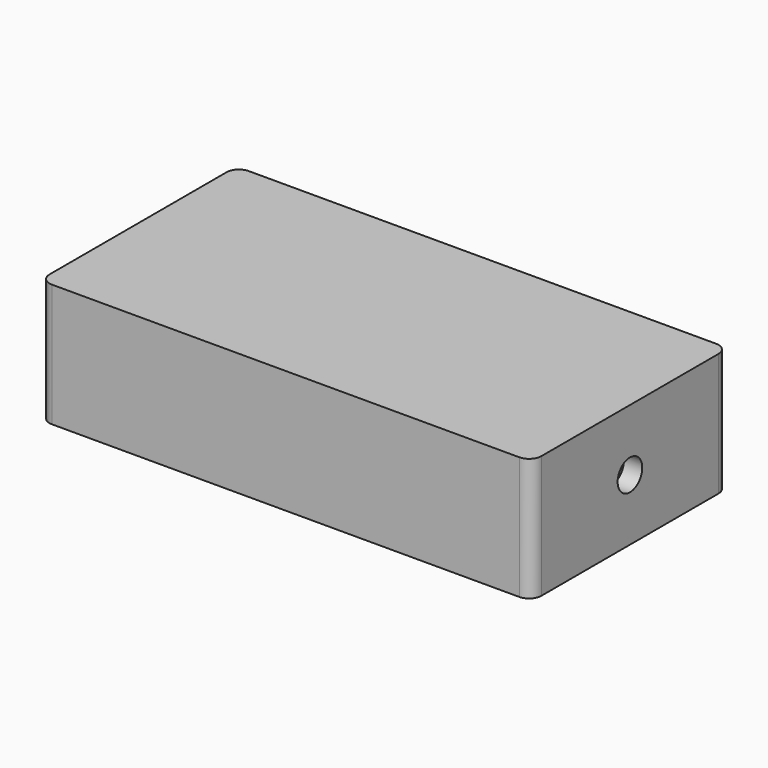
from build123d import *

# Parameters (mm, degrees)
F0_W          = 101.6
F0_H          = 50.8
F1_DEPTH      = 25.4
F2_T          = -3.81
F4_D          = 6.35
F4_DEPTH      = 12.7
F4_TIP        = 1.9077324654
F5_TEXT_SIZE  = 26.9125694306
F6_DEPTH      = 1.778
F7_W          = 93.98
F7_H          = 43.18
F7_W_2        = 88.9
F7_H_2        = 38.1
F8_DEPTH      = 21.59
F8_DEPTH_BACK = 2.54
F9_R          = 1.27
F10_R         = 2.54
F11_R         = 2.54


# Not quite as in the source:
# - Text() gives the source's letters only with a copy of the font that has no kerning and outlines rounded to 1/6400 em; it was checked with that copy


with BuildPart() as f1:
    # F0 (on Top) → F1 (new body)
    with BuildSketch(Plane.XY):
        with Locations((-25.4740342498, -0.3589369392)):
            Rectangle(F0_W, F0_H)
    extrude(amount=F1_DEPTH)

    # F2
    f2_openings = [f1.faces().sort_by_distance(p)[0] for p in [
        (-25.474034, -0.358937, 0),
    ]]
    offset(amount=F2_T, openings=f2_openings)

    # F4
    with Locations(Plane.YZ.offset(25.3259657502)):
        with Locations((-0.3589369392, 12.7)):
            Hole(F4_D / 2, depth=F4_DEPTH)
            with Locations((0, 0, -(F4_DEPTH + F4_TIP / 2))):  # 118° drill point
                Cone(0, F4_D / 2, F4_TIP, mode=Mode.SUBTRACT)

    # F5 (on face) → F6 (cut)
    with BuildSketch(Plane(origin=(0, 0, 21.59), x_dir=(1, 0, 0), z_dir=(0, 0, -1))):
        with Locations((-52.9090445489, -11.15504466)):
            Text('BOX', F5_TEXT_SIZE, font='Open Sans', text_align=(TextAlign.LEFT, TextAlign.BOTTOM))
    extrude(amount=-F6_DEPTH, mode=Mode.SUBTRACT)

    # F7 (on face) → F8 (join, two sides)
    with BuildSketch(Plane(origin=(0, 0, 0), x_dir=(1, 0, 0), z_dir=(0, 0, -1))) as f8_sk:
        with Locations((-25.4740342498, 0.3589369392)):
            Rectangle(F7_W, F7_H)
        with Locations((-25.4740342498, 0.3589369392)):
            Rectangle(F7_W_2, F7_H_2, mode=Mode.SUBTRACT)
    extrude(amount=-F8_DEPTH)
    extrude(f8_sk.sketch, amount=F8_DEPTH_BACK)

    # F9
    f9_edges = [f1.edges().sort_by_distance(p)[0] for p in [
        (21.515966, -21.948937, -1.27),
        (-72.464034, -21.948937, -1.27),
        (21.515966, 21.231063, -1.27),
        (-72.464034, 21.231063, -1.27),
        (-25.474034, -21.948937, -2.54),
        (-72.464034, -0.358937, -2.54),
        (-25.474034, 21.231063, -2.54),
        (21.515966, -0.358937, -2.54),
    ]]
    fillet(f9_edges, radius=F9_R)

    # F10
    f10_edges = [f1.edges().sort_by_distance(p)[0] for p in [
        (25.325966, -25.758937, 12.7),
    ]]
    fillet(f10_edges, radius=F10_R)

    # F11
    f11_edges = [f1.edges().sort_by_distance(p)[0] for p in [
        (-76.274034, -25.758937, 12.7),
        (-76.274034, 25.041063, 12.7),
        (25.325966, 25.041063, 12.7),
    ]]
    fillet(f11_edges, radius=F11_R)


solid = f1.part
